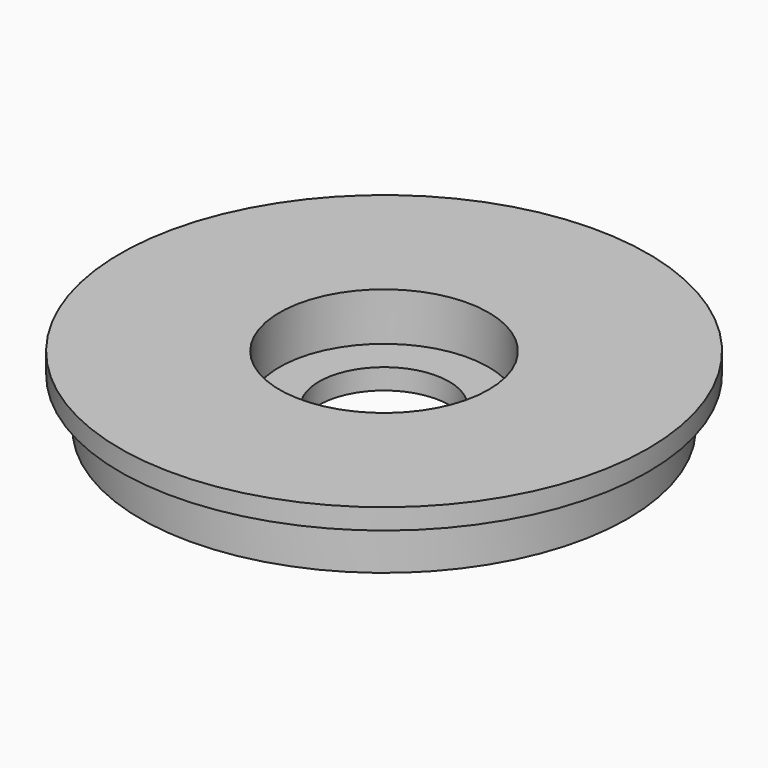
from build123d import *

# Parameters (mm, degrees)
F0_R     = 15.25
F0_R_2   = 9.5
F1_DEPTH = 3
F0_R_3   = 35.5
F2_DEPTH = 10
F3_R     = 38.5
F3_R_2   = 35.5
F4_DEPTH = 3


# Not quite as in the source:
# - a feature names something its author has since deleted; it is built from what else it names


with BuildPart() as f1:
    # F0 (on Top) → F1 (new body)
    with BuildSketch(Plane.XY):
        with Locations((-39.1464792192, 0)):
            Circle(F0_R)
        with Locations((-39.1464792192, 0)):
            Circle(F0_R_2, mode=Mode.SUBTRACT)
    extrude(amount=F1_DEPTH)


with BuildPart() as f2:
    # F0 (on Top) → F2 (new body)
    with BuildSketch(Plane.XY):
        with Locations((-39.1464792192, 0)):
            Circle(F0_R_3)
        with Locations((-39.1464792192, 0)):
            Circle(F0_R, mode=Mode.SUBTRACT)
    extrude(amount=F2_DEPTH)

    # F3 (on face) → F4 (join)
    with BuildSketch(Plane.XY.offset(10)):
        with Locations((-39.1464792192, 0)):
            Circle(F3_R)
        with Locations((-39.1464792192, 0)):
            Circle(F3_R_2, mode=Mode.SUBTRACT)
    extrude(amount=-F4_DEPTH)


solid = Compound([f1.part, f2.part])
